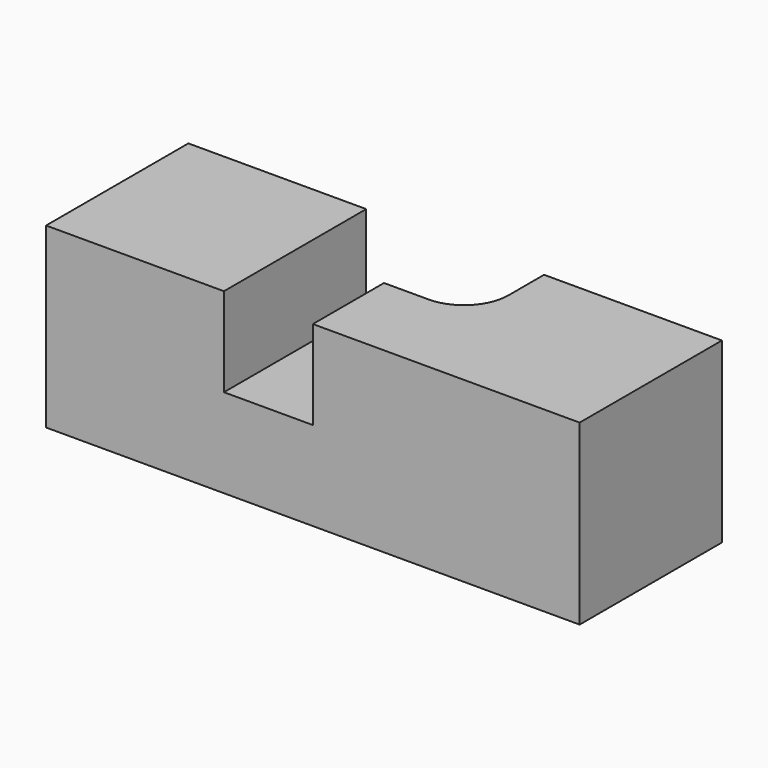
from build123d import *

# Parameters (mm, degrees)
F0_W     = 60
F0_H     = 20
F1_DEPTH = 20
F2_W     = 10
F2_H     = 20
F3_DEPTH = 10
F4_W     = 10
F4_H     = 10
F5_DEPTH = 20
F6_R     = 4.99999


# Not quite as in the source:
# - a fillet or chamfer is up to 0.001 mm smaller than in the source, because OpenCascade refuses the exact size


with BuildPart() as f1:
    # F0 (on Top) → F1 (new body)
    with BuildSketch(Plane.XY):
        with Locations((30, -10)):
            Rectangle(F0_W, F0_H)
    extrude(amount=F1_DEPTH)

    # F2 (on face) → F3 (cut)
    with BuildSketch(Plane.XY.offset(20)):
        with Locations((25, -10)):
            Rectangle(F2_W, F2_H)
    extrude(amount=-F3_DEPTH, mode=Mode.SUBTRACT)

    # F4 (on face) → F5 (cut)
    with BuildSketch(Plane.XY.offset(20)):
        with Locations((35, -5)):
            Rectangle(F4_W, F4_H)
    extrude(amount=-F5_DEPTH, mode=Mode.SUBTRACT)

    # F6 (radius 5 in the source; OpenCascade refuses exactly that, so slightly less here)
    f6_edges = [f1.edges().sort_by_distance(p)[0] for p in [
        (30, -10, 5),
        (40, -10, 10),
    ]]
    fillet(f6_edges, radius=F6_R)


solid = f1.part
